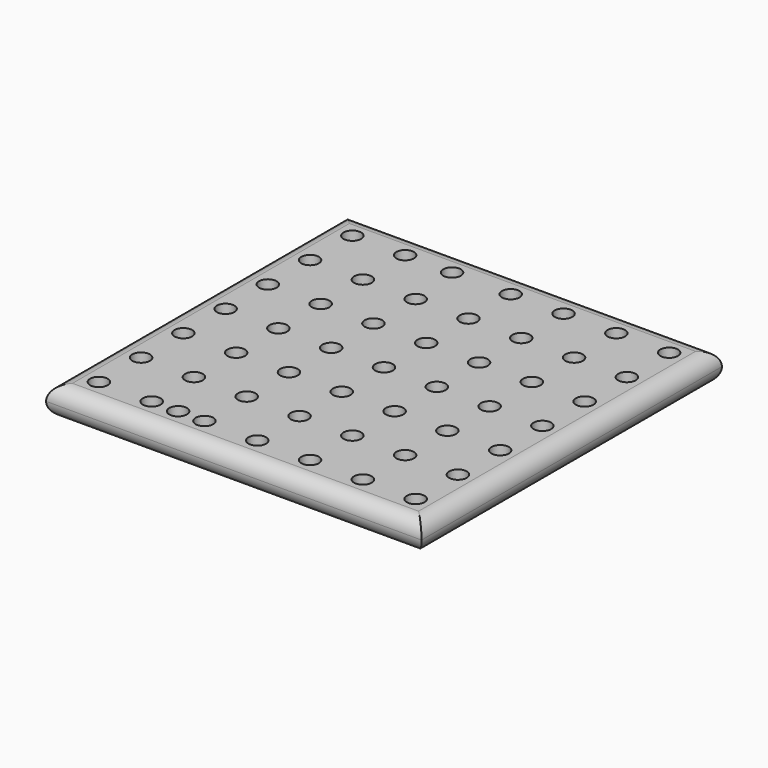
from build123d import *

# Parameters (mm, degrees)
F0_W     = 162.56
F0_H     = 162.56
F1_DEPTH = 12.7
F3_R     = 3.81
F4_DEPTH = 6.35
F5_R     = 6.34999
F6_R     = 3.81
F7_DEPTH = 6.35


# Not quite as in the source:
# - a fillet or chamfer is up to 0.001 mm smaller than in the source, because OpenCascade refuses the exact size


with BuildPart() as f1:
    # F0 (on Top) → F1 (new body)
    with BuildSketch(Plane.XY):
        with Locations((-63.3368934822, 92.4975652182)):
            Rectangle(F0_W, F0_H)
    extrude(amount=F1_DEPTH)

    # F3 (on face) → F4 (cut)
    with BuildSketch(Plane.XY.offset(12.7)):
        with Locations((-131.9168934822, 23.9175652182)):
            Circle(F3_R)
        with Locations((-86.1968934822, 23.9175652182)):
            Circle(F3_R)
        with Locations((-40.4768934822, 23.9175652182)):
            Circle(F3_R)
        with Locations((5.2431065178, 23.9175652182)):
            Circle(F3_R)
        with Locations((-109.0568934822, 23.9175652182)):
            Circle(F3_R)
        with Locations((-63.3368934822, 23.9175652182)):
            Circle(F3_R)
        with Locations((-17.6168934822, 23.9175652182)):
            Circle(F3_R)
        with Locations((-131.9168934822, 46.7775652182)):
            Circle(F3_R)
        with Locations((-131.9168934822, 69.6375652182)):
            Circle(F3_R)
        with Locations((-131.9168934822, 92.4975652182)):
            Circle(F3_R)
        with Locations((-131.9168934822, 115.3575652182)):
            Circle(F3_R)
        with Locations((-131.9168934822, 138.2175652182)):
            Circle(F3_R)
        with Locations((-131.9168934822, 161.0775652182)):
            Circle(F3_R)
        with Locations((-109.0568934822, 46.7775652182)):
            Circle(F3_R)
        with Locations((-109.0568934822, 69.6375652182)):
            Circle(F3_R)
        with Locations((-109.0568934822, 92.4975652182)):
            Circle(F3_R)
        with Locations((-109.0568934822, 115.3575652182)):
            Circle(F3_R)
        with Locations((-109.0568934822, 138.2175652182)):
            Circle(F3_R)
        with Locations((-109.0568934822, 161.0775652182)):
            Circle(F3_R)
        with Locations((-86.1968934822, 46.7775652182)):
            Circle(F3_R)
        with Locations((-63.3368934822, 46.7775652182)):
            Circle(F3_R)
        with Locations((-40.4768934822, 46.7775652182)):
            Circle(F3_R)
        with Locations((188.1231065178, 46.7775652182)):
            Circle(F3_R)
        with Locations((5.2431065178, 46.7775652182)):
            Circle(F3_R)
        with Locations((-17.6168934822, 46.7775652182)):
            Circle(F3_R)
        with Locations((-88.7368934822, 161.0775652182)):
            Circle(F3_R)
        with Locations((-86.1968934822, 138.2175652182)):
            Circle(F3_R)
        with Locations((-86.1968934822, 115.3575652182)):
            Circle(F3_R)
        with Locations((-86.1968934822, 92.4975652182)):
            Circle(F3_R)
        with Locations((-86.1968934822, 69.6375652182)):
            Circle(F3_R)
        with Locations((-63.3368934822, 69.6375652182)):
            Circle(F3_R)
        with Locations((-40.4768934822, 69.6375652182)):
            Circle(F3_R)
        with Locations((-17.6168934822, 69.6375652182)):
            Circle(F3_R)
        with Locations((5.2431065178, 69.6375652182)):
            Circle(F3_R)
        with Locations((-63.3368934822, 92.4975652182)):
            Circle(F3_R)
        with Locations((-40.4768934822, 92.4975652182)):
            Circle(F3_R)
        with Locations((-17.6168934822, 92.4975652182)):
            Circle(F3_R)
        with Locations((5.2431065178, 92.4975652182)):
            Circle(F3_R)
        with Locations((-17.6168934822, 161.0775652182)):
            Circle(F3_R)
        with Locations((-63.3368934822, 115.3575652182)):
            Circle(F3_R)
        with Locations((-63.3368934822, 161.0775652182)):
            Circle(F3_R)
        with Locations((-17.6168934822, 138.2175652182)):
            Circle(F3_R)
        with Locations((-40.4768934822, 138.2175652182)):
            Circle(F3_R)
        with Locations((-40.4768934822, 161.0775652182)):
            Circle(F3_R)
        with Locations((5.2431065178, 115.3575652182)):
            Circle(F3_R)
        with Locations((5.2431065178, 138.2175652182)):
            Circle(F3_R)
        with Locations((-40.4768934822, 115.3575652182)):
            Circle(F3_R)
        with Locations((-63.3368934822, 138.2175652182)):
            Circle(F3_R)
        with Locations((5.2431065178, 161.0775652182)):
            Circle(F3_R)
        with Locations((-17.6168934822, 115.3575652182)):
            Circle(F3_R)
    extrude(amount=-F4_DEPTH, mode=Mode.SUBTRACT)

    # F5 (radius 6.35 in the source; OpenCascade refuses exactly that, so slightly less here)
    f5_edges = [f1.edges().sort_by_distance(p)[0] for p in [
        (-144.616893, 92.497565, 12.7),
        (-144.616893, 92.497565, 0),
        (-63.336893, 173.777565, 12.7),
        (-63.336893, 173.777565, 0),
        (-63.336893, 11.217565, 12.7),
        (-63.336893, 11.217565, 0),
        (17.943107, 92.497565, 12.7),
        (17.943107, 92.497565, 0),
    ]]
    fillet(f5_edges, radius=F5_R)

    # F6 (on face) → F7 (cut)
    with BuildSketch(Plane.XY.offset(12.7)):
        with Locations((-97.6268934822, 23.9175652182)):
            Circle(F6_R)
    extrude(amount=-F7_DEPTH, mode=Mode.SUBTRACT)


solid = f1.part
